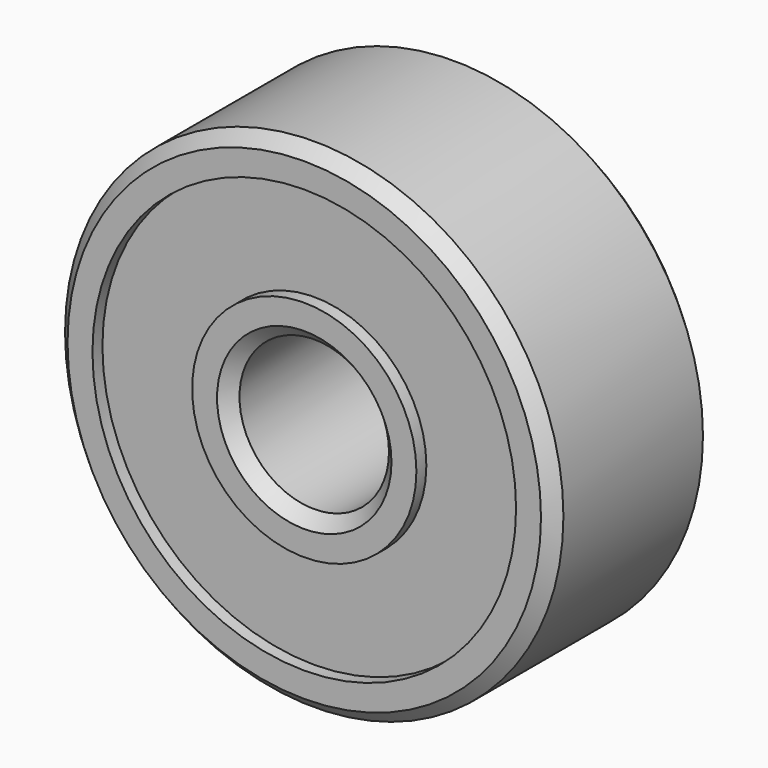
from build123d import *

# Parameters (mm, degrees)
F0_R          = 5
F0_R_2        = 1.5
F1_DEPTH      = 3.5
F2_R          = 5
F2_R_2        = 4.25
F2_R_3        = 2.25
F2_R_4        = 1.5
F3_DEPTH      = 0.25
F3_DEPTH_BACK = 3.75
F4_SIZE       = 0.24999


# Not quite as in the source:
# - a fillet or chamfer is up to 0.001 mm smaller than in the source, because OpenCascade refuses the exact size


with BuildPart() as f1:
    # F0 (on Front) → F1 (new body)
    with BuildSketch(Plane.XZ):
        Circle(F0_R)
        Circle(F0_R_2, mode=Mode.SUBTRACT)
    extrude(amount=F1_DEPTH)

    # F2 (on face) → F3 (join, two sides)
    with BuildSketch(Plane.XZ.offset(3.5)) as f3_sk:
        Circle(F2_R)
        Circle(F2_R_2, mode=Mode.SUBTRACT)
        Circle(F2_R_3)
        Circle(F2_R_4, mode=Mode.SUBTRACT)
    extrude(amount=F3_DEPTH)
    extrude(f3_sk.sketch, amount=-F3_DEPTH_BACK)

    # F4 (size 0.25 in the source; OpenCascade refuses exactly that, so slightly less here)
    f4_edges = [f1.edges().sort_by_distance(p)[0] for p in [
        (-5, -3.75, 0),
        (-1.5, -3.75, 0),
        (-1.5, 0.25, 0),
        (-5, 0.25, 0),
    ]]
    chamfer(f4_edges, length=F4_SIZE)


solid = f1.part
